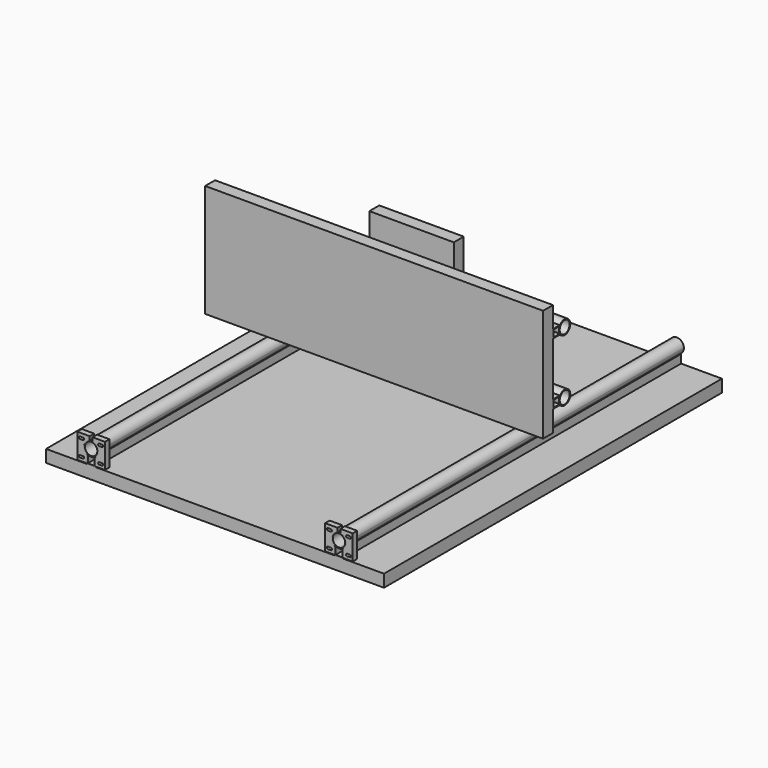
from build123d import *

# Parameters (mm, degrees)
F0_W      = 600
F0_H      = 750
F1_DEPTH  = 22
F3_DEPTH  = 750
F2_R      = 11
F5_DEPTH  = 10
F6_W      = 600
F6_H      = 200
F7_DEPTH  = 22
F8_R      = 11
F9_DEPTH  = 600
F10_W     = 22
F10_H     = 200
F11_DEPTH = 75


with BuildPart() as f1:
    # F0 (on Top) → F1 (new body)
    with BuildSketch(Plane.XY):
        Rectangle(F0_W, F0_H)
    extrude(amount=F1_DEPTH)


with BuildPart() as f3:
    # F2 (on face) → F3 (new body, through all)
    with BuildSketch(Plane.XZ.offset(375)):
        Polygon((-226, 37), (-227.5, 37), (-227.5, 22), (-212.5, 22), (-212.5, 37), (-214, 37), (-214, 23.5), (-226, 23.5), align=None)
    extrude(amount=-F3_DEPTH)


with BuildPart() as f3b:
    # F2 (on face) → F3, piece 2 (new body, through all)
    with BuildSketch(Plane.XZ.offset(375)):
        with BuildLine():
            ThreePointArc((-207.5, 47.9658560997), (-226.373774392, 58.7187626835), (-226, 37))
            ThreePointArc((-226, 37), (-220, 35.4658560997), (-214, 37))
            ThreePointArc((-214, 37), (-209.2470934162, 41.5920817077), (-207.5, 47.9658560997))
        make_face()
        with Locations((-220, 47.9658560997)):
            Circle(F2_R, mode=Mode.SUBTRACT)
    extrude(amount=-F3_DEPTH)


with BuildPart() as f3c:
    # F2 (on face) → F3, piece 3 (new body, through all)
    with BuildSketch(Plane.XZ.offset(375)):
        Polygon((212.5, 37), (212.5, 22), (227.5, 22), (227.5, 37), (226, 37), (226, 23.5), (214, 23.5), (214, 37), align=None)
    extrude(amount=-F3_DEPTH)


with BuildPart() as f3d:
    # F2 (on face) → F3, piece 4 (new body, through all)
    with BuildSketch(Plane.XZ.offset(375)):
        with BuildLine():
            ThreePointArc((232.5, 47.9658560997), (213.626225608, 58.7187626835), (214, 37))
            ThreePointArc((214, 37), (220, 35.4658560997), (226, 37))
            ThreePointArc((226, 37), (230.7529065838, 41.5920817077), (232.5, 47.9658560997))
        make_face()
        with Locations((220, 47.9658560997)):
            Circle(F2_R, mode=Mode.SUBTRACT)
    extrude(amount=-F3_DEPTH)


with BuildPart() as f5:
    # F4 (on face) → F5 (new body)
    with BuildSketch(Plane.XZ.offset(375)):
        with BuildLine():
            ThreePointArc((-227.5, 57.9658560997), (-225.1247201319, 59.3670509305), (-222.5, 60.2133048136))
            Line((-222.5, 60.2133048136), (-222.5, 67))
            Line((-222.5, 67), (-244.5, 67))
            Line((-244.5, 67), (-244.5, 23))
            Line((-244.5, 23), (-227.5, 23))
            Line((-227.5, 23), (-227.5, 37))
            Line((-227.5, 37), (-227.5, 37.9658560997))
            ThreePointArc((-227.5, 37.9658560997), (-232.5, 47.9658560997), (-227.5, 57.9658560997))
        make_face()
        with BuildLine():
            Line((-234.5, 28), (-239.5, 28))
            ThreePointArc((-239.5, 28), (-241.5, 30), (-239.5, 32))
            Line((-239.5, 32), (-234.5, 32))
            ThreePointArc((-234.5, 32), (-232.5, 30), (-234.5, 28))
        make_face(mode=Mode.SUBTRACT)
        with BuildLine():
            ThreePointArc((-239.5, 57), (-241.5, 59), (-239.5, 61))
            Line((-239.5, 61), (-234.5, 61))
            ThreePointArc((-234.5, 61), (-232.5, 59), (-234.5, 57))
            Line((-234.5, 57), (-239.5, 57))
        make_face(mode=Mode.SUBTRACT)
    extrude(amount=-F5_DEPTH)


with BuildPart() as f5b:
    # F4 (on face) → F5, piece 2 (new body)
    with BuildSketch(Plane.XZ.offset(375)):
        with BuildLine():
            Line((-217.5, 67), (-217.5, 60.2133048136))
            ThreePointArc((-217.5, 60.2133048136), (-214.8752798681, 59.3670509305), (-212.5, 57.9658560997))
            ThreePointArc((-212.5, 57.9658560997), (-208.8196601125, 53.5560260435), (-207.5, 47.9658560997))
            ThreePointArc((-207.5, 47.9658560997), (-208.8196601125, 42.375686156), (-212.5, 37.9658560997))
            Line((-212.5, 37.9658560997), (-212.5, 37))
            Line((-212.5, 37), (-212.5, 23))
            Line((-212.5, 23), (-195.5, 23))
            Line((-195.5, 23), (-195.5, 67))
            Line((-195.5, 67), (-217.5, 67))
        make_face()
        with BuildLine():
            Line((-205.5, 32), (-200.5, 32))
            ThreePointArc((-200.5, 32), (-198.5, 30), (-200.5, 28))
            Line((-200.5, 28), (-205.5, 28))
            ThreePointArc((-205.5, 28), (-207.5, 30), (-205.5, 32))
        make_face(mode=Mode.SUBTRACT)
        with BuildLine():
            ThreePointArc((-200.5, 61), (-198.5, 59), (-200.5, 57))
            Line((-200.5, 57), (-205.5, 57))
            ThreePointArc((-205.5, 57), (-207.5, 59), (-205.5, 61))
            Line((-205.5, 61), (-200.5, 61))
        make_face(mode=Mode.SUBTRACT)
    extrude(amount=-F5_DEPTH)


with BuildPart() as f5c:
    # F4 (on face) → F5, piece 3 (new body)
    with BuildSketch(Plane.XZ.offset(375)):
        with BuildLine():
            Line((195.5, 67), (195.5, 23))
            Line((195.5, 23), (212.5, 23))
            Line((212.5, 23), (212.5, 37))
            Line((212.5, 37), (212.5, 37.9658560997))
            ThreePointArc((212.5, 37.9658560997), (207.5, 47.9658560997), (212.5, 57.9658560997))
            ThreePointArc((212.5, 57.9658560997), (214.8752798681, 59.3670509305), (217.5, 60.2133048136))
            Line((217.5, 60.2133048136), (217.5, 67))
            Line((217.5, 67), (195.5, 67))
        make_face()
        with BuildLine():
            Line((205.5, 28), (200.5, 28))
            ThreePointArc((200.5, 28), (198.5, 30), (200.5, 32))
            Line((200.5, 32), (205.5, 32))
            ThreePointArc((205.5, 32), (207.5, 30), (205.5, 28))
        make_face(mode=Mode.SUBTRACT)
        with BuildLine():
            ThreePointArc((200.5, 57), (198.5, 59), (200.5, 61))
            Line((200.5, 61), (205.5, 61))
            ThreePointArc((205.5, 61), (207.5, 59), (205.5, 57))
            Line((205.5, 57), (200.5, 57))
        make_face(mode=Mode.SUBTRACT)
    extrude(amount=-F5_DEPTH)


with BuildPart() as f5d:
    # F4 (on face) → F5, piece 4 (new body)
    with BuildSketch(Plane.XZ.offset(375)):
        with BuildLine():
            Line((227.5, 37), (227.5, 23))
            Line((227.5, 23), (244.5, 23))
            Line((244.5, 23), (244.5, 67))
            Line((244.5, 67), (222.5, 67))
            Line((222.5, 67), (222.5, 60.2133048136))
            ThreePointArc((222.5, 60.2133048136), (225.1247201319, 59.3670509305), (227.5, 57.9658560997))
            ThreePointArc((227.5, 57.9658560997), (231.1803398875, 53.5560260435), (232.5, 47.9658560997))
            ThreePointArc((232.5, 47.9658560997), (231.1803398875, 42.375686156), (227.5, 37.9658560997))
            Line((227.5, 37.9658560997), (227.5, 37))
        make_face()
        with BuildLine():
            ThreePointArc((239.5, 32), (241.5, 30), (239.5, 28))
            Line((239.5, 28), (234.5, 28))
            ThreePointArc((234.5, 28), (232.5, 30), (234.5, 32))
            Line((234.5, 32), (239.5, 32))
        make_face(mode=Mode.SUBTRACT)
        with BuildLine():
            Line((239.5, 57), (234.5, 57))
            ThreePointArc((234.5, 57), (232.5, 59), (234.5, 61))
            Line((234.5, 61), (239.5, 61))
            ThreePointArc((239.5, 61), (241.5, 59), (239.5, 57))
        make_face(mode=Mode.SUBTRACT)
    extrude(amount=-F5_DEPTH)


with BuildPart() as f7:
    # F6 (on Front) → F7 (new body)
    with BuildSketch(Plane.XZ):
        with Locations((0, 189.4764214754)):
            Rectangle(F6_W, F6_H)
    extrude(amount=F7_DEPTH)


with BuildPart() as f9:
    # F8 (on face) → F9 (new body, through all)
    with BuildSketch(Plane.YZ.offset(300)):
        with BuildLine():
            ThreePointArc((38.4658560997, 244.4764214754), (29.0623701683, 256.5868137326), (15, 250.4764214754))
            ThreePointArc((15, 250.4764214754), (13.4658560997, 244.4764214754), (15, 238.4764214754))
            ThreePointArc((15, 238.4764214754), (29.0623701683, 232.3660292182), (38.4658560997, 244.4764214754))
        make_face()
        with Locations((25.9658560997, 244.4764214754)):
            Circle(F8_R, mode=Mode.SUBTRACT)
    extrude(amount=-F9_DEPTH)


with BuildPart() as f9b:
    # F8 (on face) → F9, piece 2 (new body, through all)
    with BuildSketch(Plane.YZ.offset(300)):
        Polygon((0, 251.9764214754), (0, 244.4764214754), (0, 236.9764214754), (15, 236.9764214754), (15, 238.4764214754), (1.5, 238.4764214754), (1.5, 244.4764214754), (1.5, 250.4764214754), (15, 250.4764214754), (15, 251.9764214754), align=None)
    extrude(amount=-F9_DEPTH)


with BuildPart() as f9c:
    # F8 (on face) → F9, piece 3 (new body, through all)
    with BuildSketch(Plane.YZ.offset(300)):
        Polygon((15, 141.9764214754), (0, 141.9764214754), (0, 134.4764214754), (0, 126.9764214754), (15, 126.9764214754), (15, 128.4764214754), (1.5, 128.4764214754), (1.5, 134.4764214754), (1.5, 140.4764214754), (15, 140.4764214754), align=None)
    extrude(amount=-F9_DEPTH)


with BuildPart() as f9d:
    # F8 (on face) → F9, piece 4 (new body, through all)
    with BuildSketch(Plane.YZ.offset(300)):
        with BuildLine():
            ThreePointArc((38.4658560997, 134.4764214754), (29.0623701683, 146.5868137326), (15, 140.4764214754))
            ThreePointArc((15, 140.4764214754), (13.4658560997, 134.4764214754), (15, 128.4764214754))
            ThreePointArc((15, 128.4764214754), (29.0623701683, 122.3660292182), (38.4658560997, 134.4764214754))
        make_face()
        with Locations((25.9658560997, 134.4764214754)):
            Circle(F8_R, mode=Mode.SUBTRACT)
    extrude(amount=-F9_DEPTH)


with BuildPart() as f11:
    # F10 (on Right) → F11 (new body, symmetric)
    with BuildSketch(Plane.YZ):
        with Locations((72.2158560997, 189.4764214754)):
            Rectangle(F10_W, F10_H)
    extrude(amount=F11_DEPTH, both=True)


solid = Compound([f1.part, f3.part, f3b.part, f3c.part, f3d.part, f5.part, f5b.part, f5c.part, f5d.part, f7.part, f9.part, f9b.part, f9c.part, f9d.part, f11.part])
